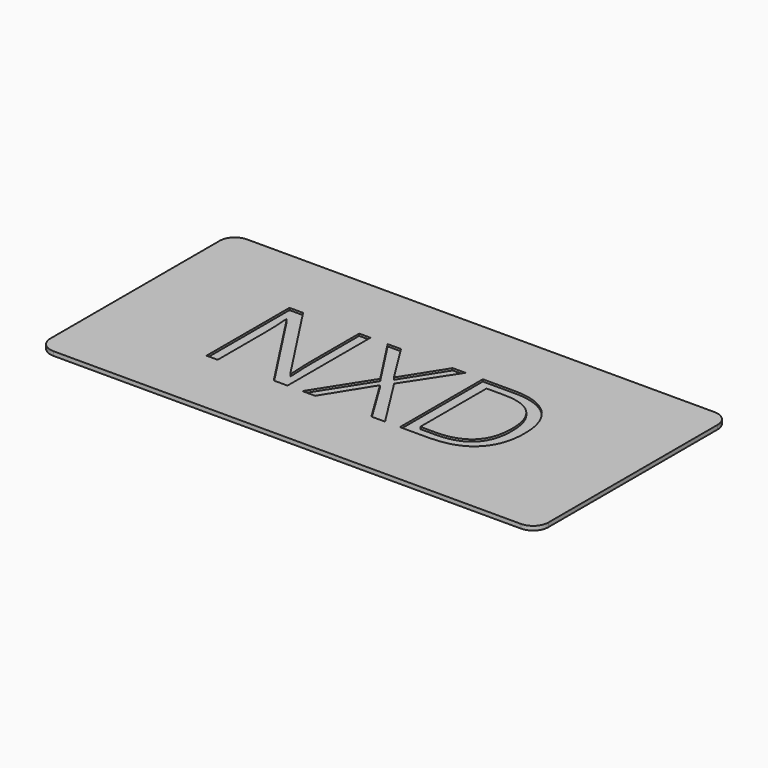
from build123d import *

# Parameters (mm, degrees)
F0_W         = 72
F0_H         = 35
F1_DEPTH     = 0.6
F2_TEXT_SIZE = 21.0018382253
F3_DEPTH     = 0.3
F4_R         = 2.2


# Not quite as in the source:
# - Text() gives the source's letters only with a copy of the font that has no kerning and outlines rounded to 1/6400 em; it was checked with that copy


with BuildPart() as f1:
    # F0 (on Top) → F1 (new body)
    with BuildSketch(Plane.XY):
        Rectangle(F0_W, F0_H)
    extrude(amount=F1_DEPTH)

    # F2 (on face) → F3 (cut)
    with BuildSketch(Plane.XY.offset(0.6)):
        with Locations((-21.6729125873, -7.5606617611)):
            Text('NXD', F2_TEXT_SIZE, font='Open Sans', text_align=(TextAlign.LEFT, TextAlign.BOTTOM))
    extrude(amount=-F3_DEPTH, mode=Mode.SUBTRACT)

    # F4
    f4_edges = [f1.edges().sort_by_distance(p)[0] for p in [
        (-36, -17.5, 0.3),
        (36, -17.5, 0.3),
        (36, 17.5, 0.3),
        (-36, 17.5, 0.3),
    ]]
    fillet(f4_edges, radius=F4_R)


solid = f1.part
